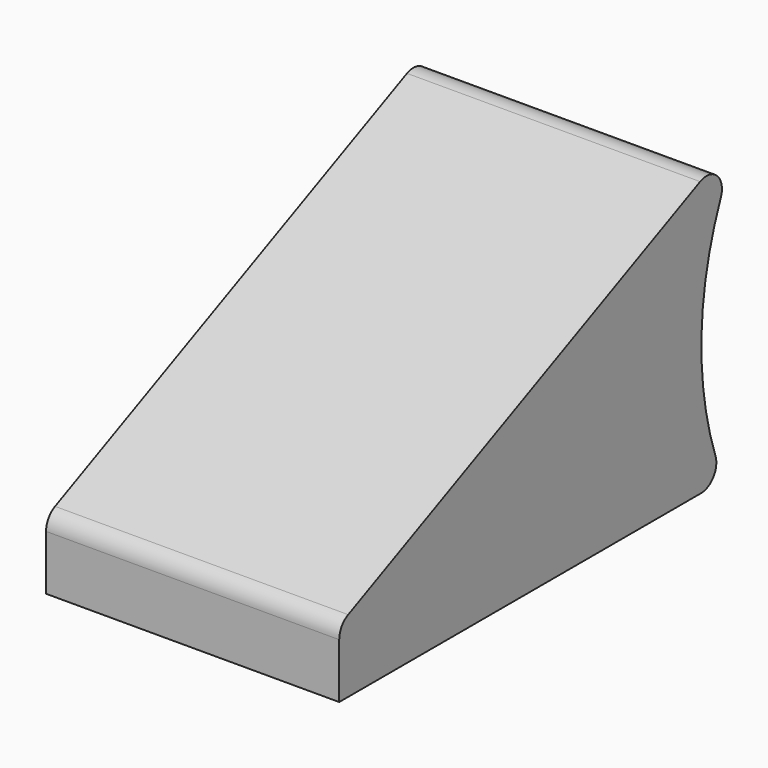
from build123d import *

# Parameters (mm, degrees)
F1_DEPTH = 30.5
F2_R     = 2
F3_R     = 2


with BuildPart() as f1:
    # F0 (on Right) → F1 (new body)
    with BuildSketch(Plane.YZ):
        with BuildLine():
            Line((0, 6.9982859343), (0, 0))
            Line((0, 0), (50, 0))
            ThreePointArc((50, 0), (47.1879454394, 15.8045232241), (52.2596416003, 31.035035469))
            Line((52.2596416003, 31.035035469), (0, 6.9982859343))
        make_face()
    extrude(amount=F1_DEPTH)

    # F2
    f2_edges = [f1.edges().sort_by_distance(p)[0] for p in [
        (15.25, 52.259642, 31.035035),
    ]]
    fillet(f2_edges, radius=F2_R)

    # F3
    f3_edges = [f1.edges().sort_by_distance(p)[0] for p in [
        (15.25, 0, 6.998286),
        (15.25, 50, 0),
    ]]
    fillet(f3_edges, radius=F3_R)


solid = f1.part
